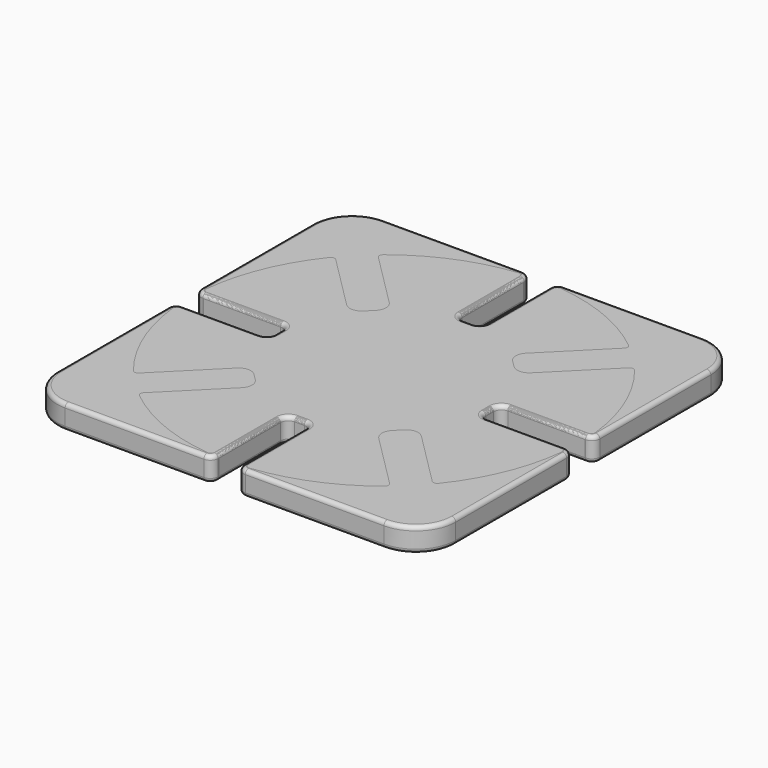
from build123d import *

# Parameters (mm, degrees)
F2_DEPTH = 3
F3_R     = 5
F4_R     = 1
F5_R     = 0.5
F7_DEPTH = 3
F8_R     = 1
F9_R     = 0.5


# Not quite as in the source:
# - a feature names something its author has since deleted; it is built from what else it names


with BuildPart() as f2:
    # F1 (on Top) → F2 (new body)
    with BuildSketch(Plane.XY):
        Polygon((1.6, -25), (25, -25), (25, -1.6), (13.25, -1.6), (13.25, 1.6), (25, 1.6), (25, 25), (1.6, 25), (1.6, 13.25), (-1.6, 13.25), (-1.6, 25), (-25, 25), (-25, 1.6), (-13.25, 1.6), (-13.25, -1.6), (-25, -1.6), (-25, -25), (-1.6, -25), (-1.6, -13.25), (1.6, -13.25), align=None)
    extrude(amount=F2_DEPTH)

    # F3
    f3_edges = [f2.edges().sort_by_distance(p)[0] for p in [
        (25, -25, 1.5),
        (-25, -25, 1.5),
        (25, 25, 1.5),
        (-25, 25, 1.5),
    ]]
    fillet(f3_edges, radius=F3_R)

    # F4
    f4_edges = [f2.edges().sort_by_distance(p)[0] for p in [
        (-1.6, -25, 1.5),
        (1.6, -25, 1.5),
        (25, -1.6, 1.5),
        (25, 1.6, 1.5),
        (-25, 1.6, 1.5),
        (-1.6, 25, 1.5),
        (1.6, 25, 1.5),
        (-25, -1.6, 1.5),
    ]]
    fillet(f4_edges, radius=F4_R)

    # F5
    f5_edges = [f2.edges().sort_by_distance(p)[0] for p in [
        (11.3, -25, 0),
        (1.892893, -24.707107, 0),
        (23.535534, -23.535534, 0),
        (1.6, -18.625, 0),
        (25, -11.3, 0),
        (0, -13.25, 0),
        (24.707107, -1.892893, 0),
        (-1.6, -18.625, 0),
        (18.625, -1.6, 0),
        (-1.892893, -24.707107, 0),
        (13.25, 0, 0),
        (-11.3, -25, 0),
        (18.625, 1.6, 0),
        (-23.535534, -23.535534, 0),
        (24.707107, 1.892893, 0),
        (-25, -11.3, 0),
        (25, 11.3, 0),
        (-24.707107, -1.892893, 0),
        (23.535534, 23.535534, 0),
        (-18.625, -1.6, 0),
        (11.3, 25, 0),
        (-13.25, 0, 0),
        (1.892893, 24.707107, 0),
        (-18.625, 1.6, 0),
        (1.6, 18.625, 0),
        (-24.707107, 1.892893, 0),
        (0, 13.25, 0),
        (-25, 11.3, 0),
        (-1.6, 18.625, 0),
        (-23.535534, 23.535534, 0),
        (-1.892893, 24.707107, 0),
        (-11.3, 25, 0),
        (11.3, -25, 3),
        (1.892893, -24.707107, 3),
        (23.535534, -23.535534, 3),
        (1.6, -18.625, 3),
        (25, -11.3, 3),
        (0, -13.25, 3),
        (24.707107, -1.892893, 3),
        (-1.6, -18.625, 3),
        (18.625, -1.6, 3),
        (-1.892893, -24.707107, 3),
        (13.25, 0, 3),
        (-11.3, -25, 3),
        (18.625, 1.6, 3),
        (-23.535534, -23.535534, 3),
        (24.707107, 1.892893, 3),
        (-25, -11.3, 3),
        (25, 11.3, 3),
        (-24.707107, -1.892893, 3),
        (23.535534, 23.535534, 3),
        (-18.625, -1.6, 3),
        (11.3, 25, 3),
        (-13.25, 0, 3),
        (1.892893, 24.707107, 3),
        (-18.625, 1.6, 3),
        (1.6, 18.625, 3),
        (-24.707107, 1.892893, 3),
        (0, 13.25, 3),
        (-25, 11.3, 3),
        (-1.6, 18.625, 3),
        (-23.535534, 23.535534, 3),
        (-1.892893, 24.707107, 3),
        (-11.3, 25, 3),
    ]]
    fillet(f5_edges, radius=F5_R)


with BuildPart() as f7:
    # F6 (on Top) → F7 (new body)
    with BuildSketch(Plane.XY):
        with BuildLine():
            Line((13.25, 1.6), (25, 1.6))
            ThreePointArc((25, 1.6), (23.1442426059, 9.5866591782), (18.8090403796, 16.5462986798))
            Line((18.8090403796, 16.5462986798), (10.5005357006, 8.2377940008))
            Line((10.5005357006, 8.2377940008), (8.2377940008, 10.5005357006))
            Line((8.2377940008, 10.5005357006), (16.5462986798, 18.8090403796))
            ThreePointArc((16.5462986798, 18.8090403796), (9.5866591782, 23.1442426059), (1.6, 25))
            Line((1.6, 25), (1.6, 13.25))
            Line((1.6, 13.25), (-1.6, 13.25))
            Line((-1.6, 13.25), (-1.6, 25))
            ThreePointArc((-1.6, 25), (-9.5866591782, 23.1442426059), (-16.5462986798, 18.8090403796))
            Line((-16.5462986798, 18.8090403796), (-8.2377940008, 10.5005357006))
            Line((-8.2377940008, 10.5005357006), (-10.5005357006, 8.2377940008))
            Line((-10.5005357006, 8.2377940008), (-18.8090403796, 16.5462986798))
            ThreePointArc((-18.8090403796, 16.5462986798), (-23.1442426059, 9.5866591782), (-25, 1.6))
            Line((-25, 1.6), (-13.25, 1.6))
            Line((-13.25, 1.6), (-13.25, -1.6))
            Line((-13.25, -1.6), (-25, -1.6))
            ThreePointArc((-25, -1.6), (-23.1442426059, -9.5866591782), (-18.8090403796, -16.5462986798))
            Line((-18.8090403796, -16.5462986798), (-10.5005357006, -8.2377940008))
            Line((-10.5005357006, -8.2377940008), (-8.2377940008, -10.5005357006))
            Line((-8.2377940008, -10.5005357006), (-16.5462986798, -18.8090403796))
            ThreePointArc((-16.5462986798, -18.8090403796), (-9.5866591782, -23.1442426059), (-1.6, -25))
            Line((-1.6, -25), (-1.6, -13.25))
            Line((-1.6, -13.25), (1.6, -13.25))
            Line((1.6, -13.25), (1.6, -25))
            ThreePointArc((1.6, -25), (9.5866591782, -23.1442426059), (16.5462986798, -18.8090403796))
            Line((16.5462986798, -18.8090403796), (8.2377940008, -10.5005357006))
            Line((8.2377940008, -10.5005357006), (10.5005357006, -8.2377940008))
            Line((10.5005357006, -8.2377940008), (18.8090403796, -16.5462986798))
            ThreePointArc((18.8090403796, -16.5462986798), (23.1442426059, -9.5866591782), (25, -1.6))
            Line((25, -1.6), (13.25, -1.6))
            Line((13.25, -1.6), (13.25, 1.6))
        make_face()
    extrude(amount=F7_DEPTH)

    # F8
    f8_edges = [f7.edges().sort_by_distance(p)[0] for p in [
        (-8.237794, 10.500536, 1.5),
        (1.6, 13.25, 1.5),
        (-8.237794, -10.500536, 1.5),
        (-13.25, -1.6, 1.5),
        (-16.546299, 18.80904, 1.5),
        (-18.80904, 16.546299, 1.5),
        (-25, 1.6, 1.5),
        (-25, -1.6, 1.5),
        (-18.80904, -16.546299, 1.5),
        (-16.546299, -18.80904, 1.5),
        (18.80904, -16.546299, 1.5),
        (25, -1.6, 1.5),
        (-1.6, 25, 1.5),
        (1.6, 25, 1.5),
        (18.80904, 16.546299, 1.5),
        (16.546299, 18.80904, 1.5),
        (8.237794, 10.500536, 1.5),
        (-1.6, 13.25, 1.5),
        (13.25, -1.6, 1.5),
        (8.237794, -10.500536, 1.5),
        (16.546299, -18.80904, 1.5),
        (25, 1.6, 1.5),
        (-1.6, -25, 1.5),
        (-1.6, -13.25, 1.5),
        (1.6, -25, 1.5),
        (-10.500536, -8.237794, 1.5),
        (-13.25, 1.6, 1.5),
        (10.500536, -8.237794, 1.5),
        (-10.500536, 8.237794, 1.5),
        (10.500536, 8.237794, 1.5),
        (13.25, 1.6, 1.5),
        (1.6, -13.25, 1.5),
    ]]
    fillet(f8_edges, radius=F8_R)

    # F9
    f9_edges = [f7.edges().sort_by_distance(p)[0] for p in [
        (23.144243, -9.586659, 3),
        (18.799674, -16.067121, 3),
        (24.654547, -1.932206, 3),
        (14.623039, -12.360298, 3),
        (19.0801, -1.6, 3),
        (10.500536, -8.652008, 3),
        (13.542893, -1.307107, 3),
        (9.369165, -9.369165, 3),
        (13.25, 0, 3),
        (8.652008, -10.500536, 3),
        (13.542893, 1.307107, 3),
        (12.360298, -14.623039, 3),
        (19.0801, 1.6, 3),
        (16.067121, -18.799674, 3),
        (24.654547, 1.932206, 3),
        (9.586659, -23.144243, 3),
        (23.144243, 9.586659, 3),
        (1.932206, -24.654547, 3),
        (18.799674, 16.067121, 3),
        (1.6, -19.0801, 3),
        (14.623039, 12.360298, 3),
        (1.307107, -13.542893, 3),
        (10.500536, 8.652008, 3),
        (0, -13.25, 3),
        (9.369165, 9.369165, 3),
        (-1.307107, -13.542893, 3),
        (8.652008, 10.500536, 3),
        (-1.6, -19.0801, 3),
        (12.360298, 14.623039, 3),
        (-1.932206, -24.654547, 3),
        (16.067121, 18.799674, 3),
        (-9.586659, -23.144243, 3),
        (9.586659, 23.144243, 3),
        (-16.067121, -18.799674, 3),
        (1.932206, 24.654547, 3),
        (-12.360298, -14.623039, 3),
        (1.6, 19.0801, 3),
        (-8.652008, -10.500536, 3),
        (1.307107, 13.542893, 3),
        (-9.369165, -9.369165, 3),
        (0, 13.25, 3),
        (-10.500536, -8.652008, 3),
        (-1.307107, 13.542893, 3),
        (-14.623039, -12.360298, 3),
        (-1.6, 19.0801, 3),
        (-18.799674, -16.067121, 3),
        (-1.932206, 24.654547, 3),
        (-23.144243, -9.586659, 3),
        (-9.586659, 23.144243, 3),
        (-24.654547, -1.932206, 3),
        (-16.067121, 18.799674, 3),
        (-19.0801, -1.6, 3),
        (-12.360298, 14.623039, 3),
        (-13.542893, -1.307107, 3),
        (-8.652008, 10.500536, 3),
        (-13.25, 0, 3),
        (-9.369165, 9.369165, 3),
        (-13.542893, 1.307107, 3),
        (-10.500536, 8.652008, 3),
        (-19.0801, 1.6, 3),
        (-14.623039, 12.360298, 3),
        (-24.654547, 1.932206, 3),
        (-18.799674, 16.067121, 3),
        (-23.144243, 9.586659, 3),
        (23.144243, -9.586659, 0),
        (18.799674, -16.067121, 0),
        (24.654547, -1.932206, 0),
        (14.623039, -12.360298, 0),
        (19.0801, -1.6, 0),
        (10.500536, -8.652008, 0),
        (13.542893, -1.307107, 0),
        (9.369165, -9.369165, 0),
        (13.25, 0, 0),
        (8.652008, -10.500536, 0),
        (13.542893, 1.307107, 0),
        (12.360298, -14.623039, 0),
        (19.0801, 1.6, 0),
        (16.067121, -18.799674, 0),
        (24.654547, 1.932206, 0),
        (9.586659, -23.144243, 0),
        (23.144243, 9.586659, 0),
        (1.932206, -24.654547, 0),
        (18.799674, 16.067121, 0),
        (1.6, -19.0801, 0),
        (14.623039, 12.360298, 0),
        (1.307107, -13.542893, 0),
        (10.500536, 8.652008, 0),
        (0, -13.25, 0),
        (9.369165, 9.369165, 0),
        (-1.307107, -13.542893, 0),
        (8.652008, 10.500536, 0),
        (-1.6, -19.0801, 0),
        (12.360298, 14.623039, 0),
        (-1.932206, -24.654547, 0),
        (16.067121, 18.799674, 0),
        (-9.586659, -23.144243, 0),
        (9.586659, 23.144243, 0),
        (-16.067121, -18.799674, 0),
        (1.932206, 24.654547, 0),
        (-12.360298, -14.623039, 0),
        (1.6, 19.0801, 0),
        (-8.652008, -10.500536, 0),
        (1.307107, 13.542893, 0),
        (-9.369165, -9.369165, 0),
        (0, 13.25, 0),
        (-10.500536, -8.652008, 0),
        (-1.307107, 13.542893, 0),
        (-14.623039, -12.360298, 0),
        (-1.6, 19.0801, 0),
        (-18.799674, -16.067121, 0),
        (-1.932206, 24.654547, 0),
        (-23.144243, -9.586659, 0),
        (-9.586659, 23.144243, 0),
        (-24.654547, -1.932206, 0),
        (-16.067121, 18.799674, 0),
        (-19.0801, -1.6, 0),
        (-12.360298, 14.623039, 0),
        (-13.542893, -1.307107, 0),
        (-8.652008, 10.500536, 0),
        (-13.25, 0, 0),
        (-9.369165, 9.369165, 0),
        (-13.542893, 1.307107, 0),
        (-10.500536, 8.652008, 0),
        (-19.0801, 1.6, 0),
        (-14.623039, 12.360298, 0),
        (-24.654547, 1.932206, 0),
        (-18.799674, 16.067121, 0),
        (-23.144243, 9.586659, 0),
    ]]
    fillet(f9_edges, radius=F9_R)


solid = Compound([f2.part, f7.part])
